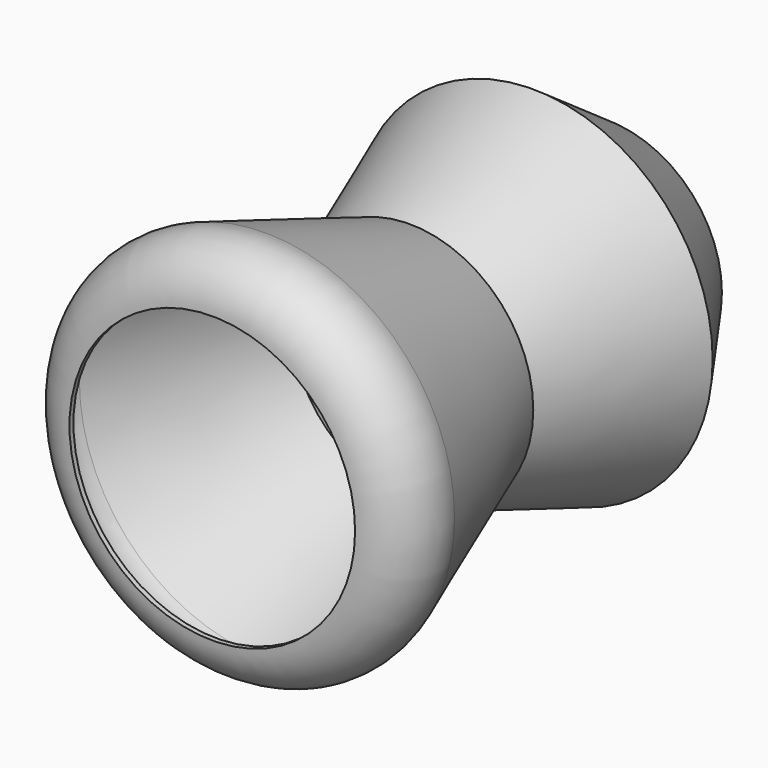
from build123d import *

# Parameters (mm, degrees)
F0_R     = 63.5
F1_DEPTH = 127
F1_TAPER = -20
F2_SIZE  = 50.8
F3_R     = 25.4
F4_T     = -2.54


# Not quite as in the source:
# - a shell that OpenCascade refuses in one call is made with other operations: the cavity is built on its own and cut out


with BuildPart() as f1:
    # F0 (on Front) → F1 (new body, symmetric)
    with BuildSketch(Plane.XZ):
        Circle(F0_R)
    extrude(amount=F1_DEPTH, both=True, taper=F1_TAPER)

    # F2
    f2_edges = [f1.edges().sort_by_distance(p)[0] for p in [
        (-109.72422, 127, 0),
    ]]
    chamfer(f2_edges, length=F2_SIZE)

    # F3
    f3_edges = [f1.edges().sort_by_distance(p)[0] for p in [
        (-109.72422, -127, 0),
    ]]
    fillet(f3_edges, radius=F3_R)

    # F4: a shell. OpenCascade refuses it in one call, so the cavity is built on its own and cut out:
    # the body offset inwards by the wall thickness, plus a prism from it out through each open face.
    f4_core = offset(f1.part, amount=F4_T, kind=Kind.INTERSECTION, mode=Mode.PRIVATE)
    f4_exits = [f4_core.faces().sort_by_distance(p)[0] for p in [
        (0, -124.46, 0),
    ]]
    add(f4_core, mode=Mode.SUBTRACT)
    extrude(f4_exits, amount=-F4_T, mode=Mode.SUBTRACT)


solid = f1.part
